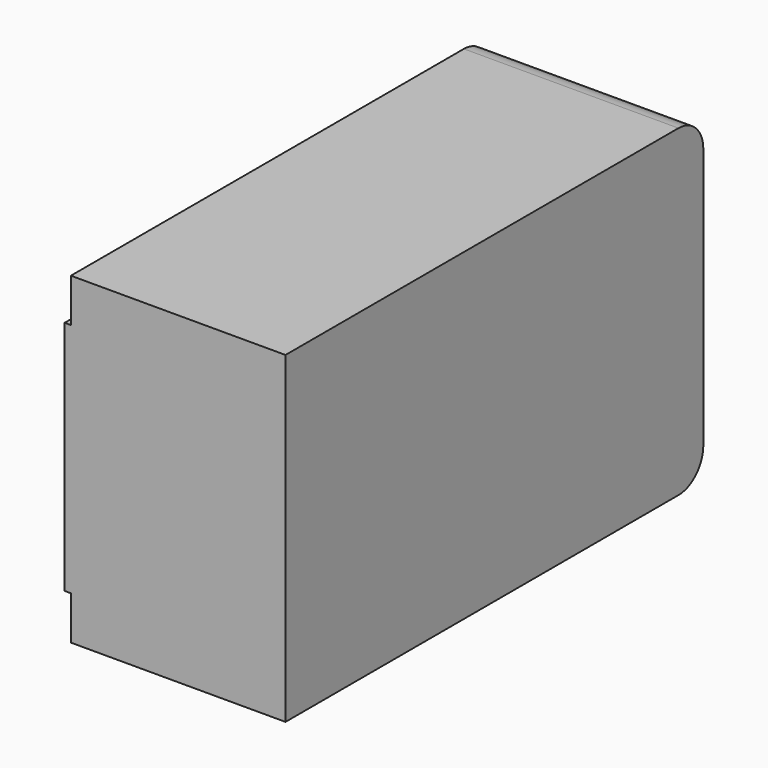
from build123d import *

# Parameters (mm, degrees)
F0_W      = 34.5459179953
F0_H      = 84.0644203126
F1_DEPTH  = 2
F2_W      = 2
F2_H      = 84.0644203126
F3_DEPTH  = 50
F4_W      = 2
F4_H      = 84.0644203126
F5_DEPTH  = 50
F6_W      = 84.0644203126
F6_H      = 2.4206031561
F7_DEPTH  = 32.2
F8_W      = 30.5459179953
F8_H      = 2
F9_DEPTH  = 47.6
F10_R     = 5
F11_R     = 5
F12_W     = 2
F12_H     = 47.5793968439
F13_DEPTH = 31.3
F14_W     = 4.5
F14_H     = 32
F15_DEPTH = 25
F16_W     = 42.5153374672
F16_H     = 38
F17_DEPTH = 1
F18_R     = 3.3259647968
F19_DEPTH = 1
F20_R     = 0.99999
F22_DEPTH = 1


# Not quite as in the source:
# - a fillet or chamfer is up to 0.001 mm smaller than in the source, because OpenCascade refuses the exact size


with BuildPart() as f1:
    # F0 (on Top) → F1 (new body)
    with BuildSketch(Plane.XY):
        with Locations((-31.5246856771, -0.4831273109)):
            Rectangle(F0_W, F0_H)
    extrude(amount=F1_DEPTH)

    # F2 (on face) → F3 (join)
    with BuildSketch(Plane.XY.offset(2)):
        with Locations((-15.2517266795, -0.4831273109)):
            Rectangle(F2_W, F2_H)
    extrude(amount=F3_DEPTH)

    # F4 (on face) → F5 (join)
    with BuildSketch(Plane.XY.offset(2)):
        with Locations((-47.7976446748, -0.4831273109)):
            Rectangle(F4_W, F4_H)
    extrude(amount=F5_DEPTH)

    # F6 (on face) → F7 (join)
    with BuildSketch(Plane.YZ.offset(-46.7976446748)):
        with Locations((-0.4831273109, 50.789698422)):
            Rectangle(F6_W, F6_H)
    extrude(amount=F7_DEPTH)

    # F8 (on face) → F9 (join)
    with BuildSketch(Plane.XY.offset(2)):
        with Locations((-31.5246856771, 40.5490828454)):
            Rectangle(F8_W, F8_H)
    extrude(amount=F9_DEPTH)

    # F10
    f10_edges = [f1.edges().sort_by_distance(p)[0] for p in [
        (-31.524686, 41.549083, 52),
    ]]
    fillet(f10_edges, radius=F10_R)

    # F11
    f11_edges = [f1.edges().sort_by_distance(p)[0] for p in [
        (-31.524686, 41.549083, 0),
    ]]
    fillet(f11_edges, radius=F11_R)

    # F12 (on face) → F13 (join)
    with BuildSketch(Plane(origin=(-16.2517266795, 0, 0), x_dir=(0, -1, 0), z_dir=(-1, 0, 0))):
        with Locations((41.5153374672, 25.789698422)):
            Rectangle(F12_W, F12_H)
    extrude(amount=F13_DEPTH)

    # F14 (on face) → F15 (cut)
    with BuildSketch(Plane(origin=(-48.7976446748, 0, 0), x_dir=(0, -1, 0), z_dir=(-1, 0, 0))):
        with Locations((-19.0076687336, 26)):
            Rectangle(F14_W, F14_H)
    extrude(amount=-F15_DEPTH, mode=Mode.SUBTRACT)

    # F16 (on face) → F17 (join)
    with BuildSketch(Plane(origin=(-48.7976446748, 0, 0), x_dir=(0, -1, 0), z_dir=(-1, 0, 0))):
        with Locations((21.2576687336, 26)):
            Rectangle(F16_W, F16_H)
    extrude(amount=F17_DEPTH)

    # F18 (on face) → F19 (join)
    with BuildSketch(Plane(origin=(-49.7976446748, 0, 0), x_dir=(0, -1, 0), z_dir=(-1, 0, 0))):
        with Locations((10.0552504882, 26)):
            Circle(F18_R)
    extrude(amount=F19_DEPTH)

    # F20 (radius 1 in the source; OpenCascade refuses exactly that, so slightly less here)
    f20_edges = [f1.edges().sort_by_distance(p)[0] for p in [
        (-50.797645, -6.729286, 26),
    ]]
    fillet(f20_edges, radius=F20_R)

    # F21 (on face) → F22 (cut)
    with BuildSketch(Plane(origin=(-50.7976446748, 0, 0), x_dir=(0, -1, 0), z_dir=(-1, 0, 0))):
        Polygon((11.3802812994, 26.4259647968), (10.0552504882, 26.4259647968), (8.548588492, 26.4259647968), (8.548588492, 25.5740352032), (11.3802812994, 25.5740352032), align=None)
    extrude(amount=-F22_DEPTH, mode=Mode.SUBTRACT)


solid = f1.part
